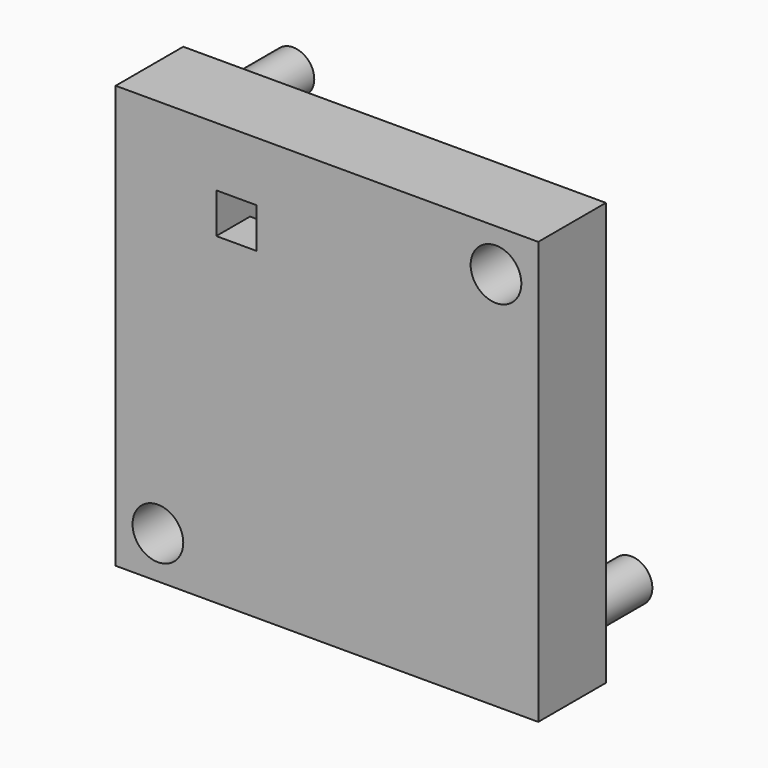
from build123d import *

# Parameters (mm, degrees)
F0_R          = 3
F0_R_2        = 2.5
F1_DEPTH      = 5
F0_W          = 4.7752
F0_H          = 4.7752
F2_DEPTH      = 5
F3_DEPTH      = 15
F3_DEPTH_BACK = 5


with BuildPart() as f1:
    # F0 (on Front) → F1 (new body, symmetric)
    with BuildSketch(Plane.XZ):
        Polygon((-25, -25), (25, -25), (25, 25), (-13.09502, 25), (-25, 25), align=None)
        with Locations((-20, -20)):
            Circle(F0_R, mode=Mode.SUBTRACT)
        with Locations((20, -20)):
            Circle(F0_R_2, mode=Mode.SUBTRACT)
        Polygon((-13.09502, 13.21694), (-13.09502, 17.97944), (-8.33252, 17.97944), (-8.33252, 13.21694), (-8.33252, 3.5414441053), (-13.09502, 3.5414441053), (-13.09502, -11.8404025305), (-4.4399380628, -11.8404025305), (6.1322724736, -11.8404025305), (6.1322724736, -2.3876), (2.3876, -2.3876), (-2.3876, -2.3876), (-2.3876, 2.3876), (2.3876, 2.3876), (6.1322724736, 2.3876), (6.1322724736, 9.5728570595), (1.8619408365, 9.5728570595), (1.8619408365, 14.3480570595), (8.9338924736, 14.3480570595), (11.5732288948, 14.3480570595), (11.5732288948, 13.8279201027), (11.5732288948, 9.2561525788), (11.5732288948, 2.3876), (11.5732288948, -2.3876), (11.5732288948, -16.6029025305), (-17.85752, -16.6029025305), (-17.85752, 3.5414441053), (-17.85752, 7.8989091825), (-13.09502, 7.8989091825), align=None, mode=Mode.SUBTRACT)
        with Locations((-20, 20)):
            Circle(F0_R_2, mode=Mode.SUBTRACT)
        with Locations((20, 20)):
            Circle(F0_R, mode=Mode.SUBTRACT)
    extrude(amount=F1_DEPTH, both=True)

    # F0 (on Front) → F2 (join)
    with BuildSketch(Plane.XZ):
        Polygon((-8.33252, 13.21694), (-13.09502, 13.21694), (-13.09502, 7.8989091825), (-17.85752, 7.8989091825), (-17.85752, 3.5414441053), (-17.85752, -16.6029025305), (11.5732288948, -16.6029025305), (11.5732288948, -2.3876), (11.5732288948, 2.3876), (11.5732288948, 9.2561525788), (11.5732288948, 13.8279201027), (11.5732288948, 14.3480570595), (8.9338924736, 14.3480570595), (1.8619408365, 14.3480570595), (1.8619408365, 9.5728570595), (6.1322724736, 9.5728570595), (6.1322724736, 2.3876), (2.3876, 2.3876), (2.3876, -2.3876), (6.1322724736, -2.3876), (6.1322724736, -11.8404025305), (-4.4399380628, -11.8404025305), (-13.09502, -11.8404025305), (-13.09502, 3.5414441053), (-8.33252, 3.5414441053), align=None)
        Rectangle(F0_W, F0_H)
    extrude(amount=F2_DEPTH)

    # F0 (on Front) → F3 (join, two sides)
    with BuildSketch(Plane.XZ) as f3_sk:
        with Locations((-20, 20)):
            Circle(F0_R_2)
        with Locations((20, -20)):
            Circle(F0_R_2)
    extrude(amount=-F3_DEPTH)
    extrude(f3_sk.sketch, amount=F3_DEPTH_BACK)


solid = f1.part
